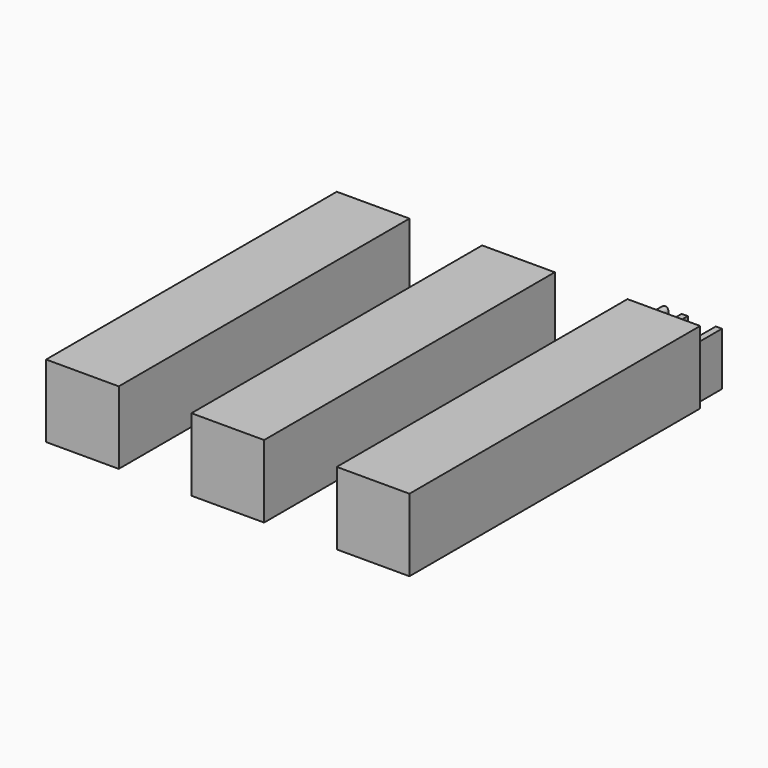
from build123d import *

# Parameters (mm, degrees)
F0_W         = 25.4
F0_H         = 25.4
F1_DEPTH     = 63.5
F2_TEXT_SIZE = 25.9846547315
F3_DEPTH     = 12.7


# Not quite as in the source:
# - Text() gives the source's letters only with a copy of the font that has no kerning and outlines rounded to 1/6400 em; it was checked with that copy


with BuildPart() as f1:
    # F0 (on Front) → F1 (new body, symmetric)
    with BuildSketch(Plane.XZ):
        with Locations((50.8, 0)):
            Rectangle(F0_W, F0_H)
    extrude(amount=F1_DEPTH, both=True)

    # F2 (on face) → F3 (join)
    with BuildSketch(Plane(origin=(0, 63.5, 0), x_dir=(-1, 0, 0), z_dir=(0, 1, 0))):
        with Locations((-63.5, -12.7)):
            Text('Hi', F2_TEXT_SIZE, font='Open Sans', text_align=(TextAlign.LEFT, TextAlign.BOTTOM))
    extrude(amount=F3_DEPTH)


with BuildPart() as f1b:
    # F0 (on Front) → F1, piece 2 (new body, symmetric)
    with BuildSketch(Plane.XZ):
        Rectangle(F0_W, F0_H)
    extrude(amount=F1_DEPTH, both=True)


with BuildPart() as f1c:
    # F0 (on Front) → F1, piece 3 (new body, symmetric)
    with BuildSketch(Plane.XZ):
        with Locations((-50.8, 0)):
            Rectangle(F0_W, F0_H)
    extrude(amount=F1_DEPTH, both=True)


solid = Compound([f1.part, f1b.part, f1c.part])
